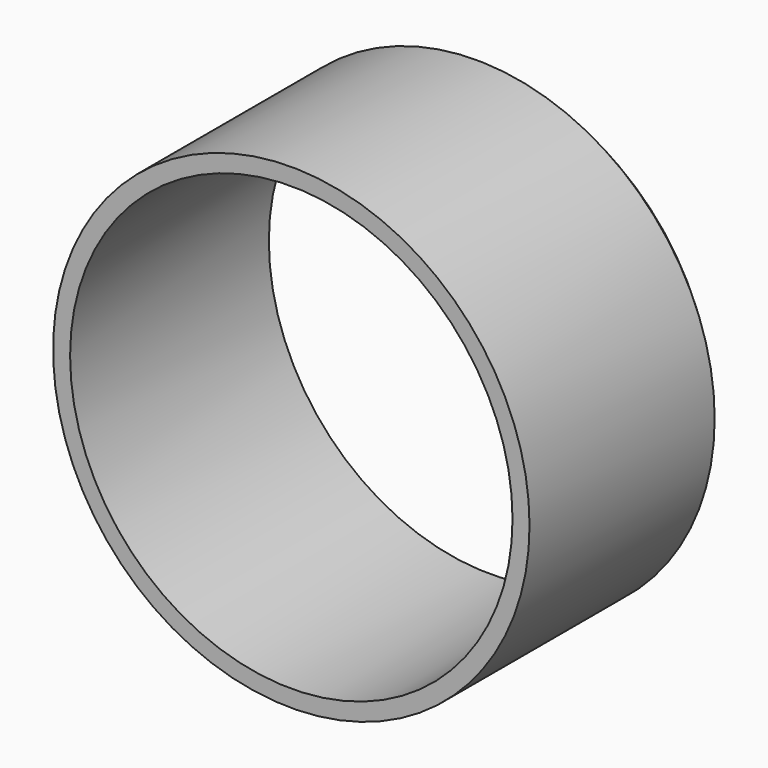
from build123d import *

# Parameters (mm, degrees)
F0_R     = 17.78
F0_R_2   = 16.51
F1_DEPTH = 19.812


# Not quite as in the source:
# - a fillet or chamfer that OpenCascade refuses, or shapes differently, is made with other operations: its cross-section is extruded or revolved along the edge and cut away or added


with BuildPart() as f1:
    # F0 (on Front) → F1 (new body)
    with BuildSketch(Plane.XZ):
        with Locations((-65.9729540348, 0)):
            Circle(F0_R)
        with Locations((-65.9729540348, 0)):
            Circle(F0_R_2, mode=Mode.SUBTRACT)
    extrude(amount=-F1_DEPTH)

    # F2: chamfer of 2.54 on 1 edges, made by hand

    # F2_s1 → F2_t2 (revolve, cut)
    with BuildSketch(Plane.XY):
        Polygon((-48.1929540348, 17.272), (-50.7329540348, 19.812), (-48.1929540348, 19.812), align=None)
    revolve(axis=Axis((-65.9729540348, 19.812, 0), (0, -1, 0)), mode=Mode.SUBTRACT)


solid = f1.part
